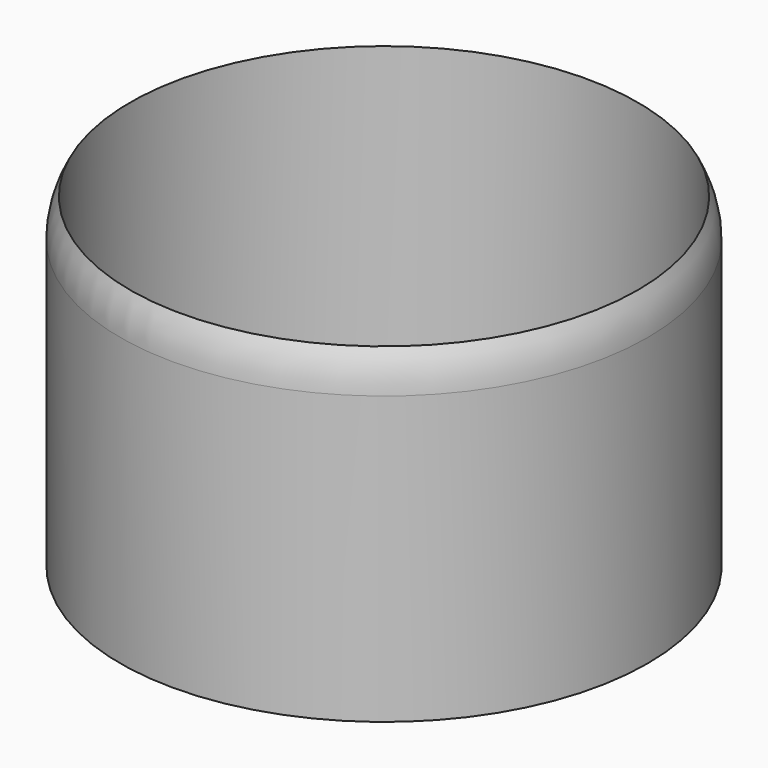
from build123d import *

# Parameters (mm, degrees)
F0_R     = 16.2
F0_R_2   = 15.6
F1_DEPTH = 20


# Not quite as in the source:
# - a fillet or chamfer that OpenCascade refuses, or shapes differently, is made with other operations: its cross-section is extruded or revolved along the edge and cut away or added
# - a feature names something its author has since deleted; it is built from what else it names


with BuildPart() as f1:
    # F0 (on Top) → F1 (new body)
    with BuildSketch(Plane.XY):
        Circle(F0_R)
        Circle(F0_R_2, mode=Mode.SUBTRACT)
    extrude(amount=F1_DEPTH)

    # F2: fillet of radius 5 on 1 edges, made by hand

    # F2_s1 → F2_t2 (revolve, cut)
    with BuildSketch(Plane.XZ):
        with BuildLine():
            ThreePointArc((16.2, 17.6251315826), (16.0476798574, 18.849876454), (15.6, 20))
            Line((15.6, 20), (16.2, 20))
            Line((16.2, 20), (16.2, 17.6251315826))
        make_face()
    revolve(axis=Axis((0, 0, 20), (0, 0, 1)), mode=Mode.SUBTRACT)


solid = f1.part
